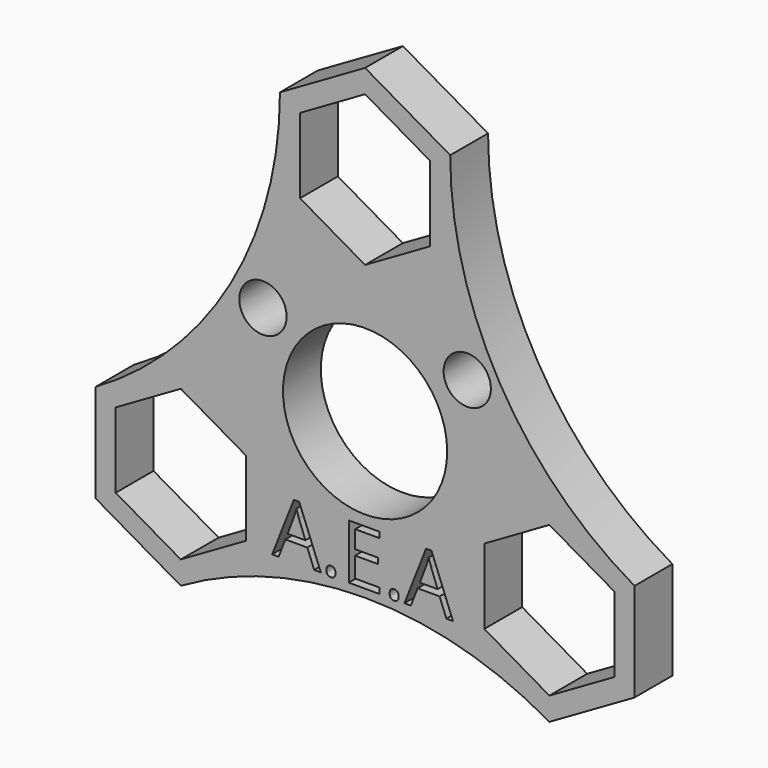
from build123d import *

# Parameters (mm, degrees)
F0_R         = 14.2875
F0_R_2       = 11.0236
F1_DEPTH     = 6.35
F2_TEXT_SIZE = 9.3304396917
F3_DEPTH     = 25.4
F4_TEXT_SIZE = 10.3171112844
F5_DEPTH     = 6.351
F6_R         = 3.1785659394
F6_R_2       = 3.175
F7_DEPTH     = 25.4


# Not quite as in the source:
# - Text() gives the source's letters only with a copy of the font that has no kerning and outlines rounded to 1/6400 em; it was checked with that copy


with BuildPart() as f1:
    # F0 (on Front) → F1 (new body)
    with BuildSketch(Plane.XZ):
        with BuildLine():
            Line((0, 15.3767728463), (-11.43, 21.9758864232))
            Line((-11.43, 21.9758864232), (-11.43, 35.1741135768))
            ThreePointArc((-11.43, 35.1741135768), (-18.0608518263, 10.4274376637), (-36.1766759131, -7.6883864232))
            Line((-36.1766759131, -7.6883864232), (-24.7466759131, -1.0892728463))
            Line((-24.7466759131, -1.0892728463), (-13.3166759131, -7.6883864232))
            Line((-13.3166759131, -7.6883864232), (-13.3166759131, -20.8866135768))
            Line((-13.3166759131, -20.8866135768), (-24.7466759131, -27.4857271537))
            ThreePointArc((-24.7466759131, -27.4857271537), (0, -20.8548753274), (24.7466759131, -27.4857271537))
            Line((24.7466759131, -27.4857271537), (13.3166759131, -20.8866135768))
            Line((13.3166759131, -20.8866135768), (13.3166759131, -7.6883864232))
            Line((13.3166759131, -7.6883864232), (24.7466759131, -1.0892728463))
            Line((24.7466759131, -1.0892728463), (36.1766759131, -7.6883864232))
            ThreePointArc((36.1766759131, -7.6883864232), (18.0608518263, 10.4274376637), (11.43, 35.1741135768))
            Line((11.43, 35.1741135768), (11.43, 21.9758864232))
            Line((11.43, 21.9758864232), (0, 15.3767728463))
        make_face()
        Circle(F0_R, mode=Mode.SUBTRACT)
        Polygon((-11.43, 35.1741135768), (-11.43, 21.9758864232), (0, 15.3767728463), (11.43, 21.9758864232), (11.43, 35.1741135768), (0, 41.7732271537), align=None)
        Polygon((0, 18.4856885759), (-8.7376, 23.5303442879), (-8.7376, 33.6196557121), (0, 38.6643114241), (8.7376, 33.6196557121), (8.7376, 23.5303442879), align=None, mode=Mode.SUBTRACT)
        Polygon((-24.7466759131, -1.0892728463), (-36.1766759131, -7.6883864232), (-36.1766759131, -20.8866135768), (-24.7466759131, -27.4857271537), (-13.3166759131, -20.8866135768), (-13.3166759131, -7.6883864232), align=None)
        Polygon((-16.0090759131, -19.3321557121), (-24.7466759131, -24.3768114241), (-33.4842759131, -19.3321557121), (-33.4842759131, -9.2428442879), (-24.7466759131, -4.1981885759), (-16.0090759131, -9.2428442879), align=None, mode=Mode.SUBTRACT)
        Polygon((36.1766759131, -20.8866135768), (36.1766759131, -7.6883864232), (24.7466759131, -1.0892728463), (13.3166759131, -7.6883864232), (13.3166759131, -20.8866135768), (24.7466759131, -27.4857271537), align=None)
        Polygon((24.7466759131, -4.1981885759), (33.4842759131, -9.2428442879), (33.4842759131, -19.3321557121), (24.7466759131, -24.3768114241), (16.0090759131, -19.3321557121), (16.0090759131, -9.2428442879), align=None, mode=Mode.SUBTRACT)
        Circle(F0_R)
        Circle(F0_R_2, mode=Mode.SUBTRACT)
    extrude(amount=F1_DEPTH)

    # F2 (on Front) → F3 (cut)
    with BuildSketch(Plane.XZ):
        with Locations((-7.5649926439, -19.9034120888)):
            Text('Abby', F2_TEXT_SIZE, font='Open Sans', text_align=(TextAlign.LEFT, TextAlign.BOTTOM))
    extrude(amount=-F3_DEPTH, mode=Mode.SUBTRACT)

    # F4 (on face) → F5 (cut, through all)
    with BuildSketch(Plane.XZ.offset(6.35)):
        with Locations((-12.4780666083, -19.7856556624)):
            Text('A.E.A', F4_TEXT_SIZE, font='Open Sans', text_align=(TextAlign.LEFT, TextAlign.BOTTOM))
    extrude(amount=-F5_DEPTH, mode=Mode.SUBTRACT)

    # F6 (on Front) → F7 (cut)
    with BuildSketch(Plane.XZ):
        with Locations((-13.716, 8.9458413422)):
            Circle(F6_R)
        with Locations((13.716, 9.3479026109)):
            Circle(F6_R_2)
    extrude(amount=F7_DEPTH, mode=Mode.SUBTRACT)


solid = f1.part
